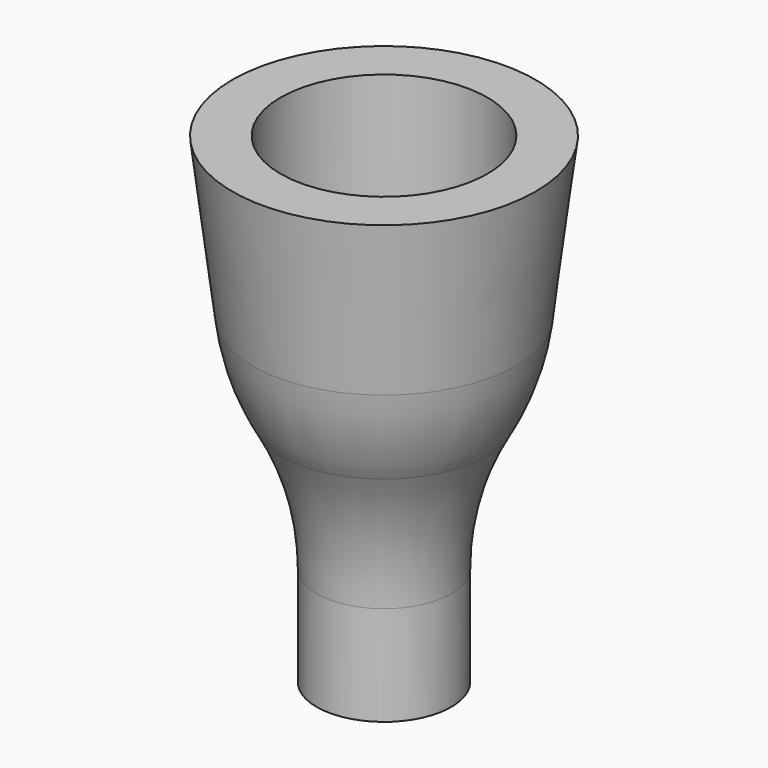
from build123d import *


# Not quite as in the source:
# - a feature names something its author has since deleted; it is built from what else it names


with BuildPart() as f1:
    # F0 (on Front) → F1 (revolve)
    with BuildSketch(Plane.XZ):
        with BuildLine():
            ThreePointArc((-21.2629083544, 48.211786896), (-15.8463196743, 34.9304531122), (-14, 20.7063762118))
            Line((-14, 20.7063762118), (-14, 0))
            Line((-14, 0), (-12, 0))
            Line((-12, 0), (-12, 43))
            Line((-12, 43), (-7.5, 43))
            Line((-7.5, 43), (-7.5, 45))
            Line((-7.5, 45), (-15, 45))
            Line((-15, 45), (-21.5, 60.9745979309))
            Line((-21.5, 60.9745979309), (-21.5, 100))
            Line((-21.5, 100), (-31.5, 100))
            Line((-31.5, 100), (-27.405355799, 66.7795249261))
            ThreePointArc((-27.405355799, 66.7795249261), (-25.2508232926, 57.1924026226), (-21.2629083544, 48.211786896))
        make_face()
    revolve(axis=Axis((0, 0, -6.6078525846), (0, 0, -1)))


solid = f1.part
